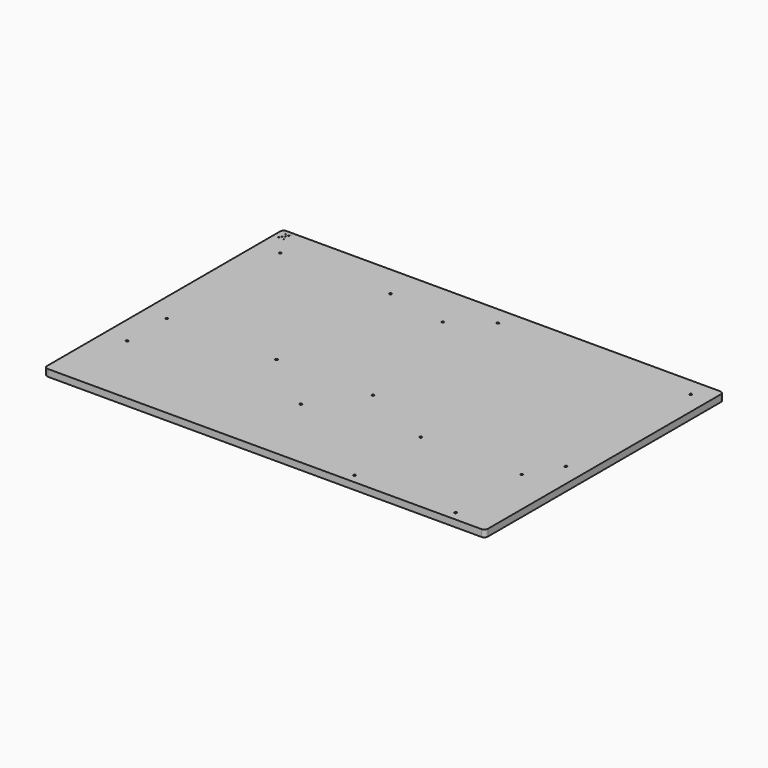
from build123d import *

# Parameters (mm, degrees)
F0_W         = 609.6
F0_H         = 412.75
F1_DEPTH     = 9.525
F2_R         = 1.5875
F3_DEPTH     = 25.4
F5_D         = 3.175
F7_D         = 3.175
F8_R         = 5.08
F9_TEXT_SIZE = 17.3569139507
F10_DEPTH    = 0.254


# Not quite as in the source:
# - Text() gives the source's letters only with a copy of the font that has no kerning and outlines rounded to 1/6400 em; it was checked with that copy


with BuildPart() as f1:
    # F0 (on Top) → F1 (new body)
    with BuildSketch(Plane.XY):
        with Locations((3.2237693667, 74.4166416769)):
            Rectangle(F0_W, F0_H)
    extrude(amount=F1_DEPTH)

    # F2 (on face) → F3 (cut)
    with BuildSketch(Plane.XY.offset(9.525)):
        with Locations((-269.8262306333, 236.3416416769)):
            Circle(F2_R)
        with Locations((-269.8262306333, 40.2536416769)):
            Circle(F2_R)
        with Locations((-270.5882306333, -27.2341583231)):
            Circle(F2_R)
        with Locations((-117.4262306333, 236.3416416769)):
            Circle(F2_R)
        with Locations((-117.4262306333, 39.4916416769)):
            Circle(F2_R)
        with Locations((-31.7012306333, -25.7101583231)):
            Circle(F2_R)
        with Locations((-32.0822306333, 220.1872416769)):
            Circle(F2_R)
    extrude(amount=-F3_DEPTH, mode=Mode.SUBTRACT)

    # F5 (through all)
    with Locations(Plane.XY.offset(9.525)):
        with Locations((117.5237693667, -4.9583583231), (257.2237693667, -4.9583583231), (257.2237693667, -119.2583583231), (117.5237693667, -119.2583583231)):
            Hole(F5_D / 2)

    # F7 (through all)
    with Locations(Plane.XY.offset(9.525)):
        with Locations((15.9237693667, 255.3916416769), (282.6237693667, 255.3916416769), (282.6237693667, 39.4916416769), (15.9237693667, 39.4916416769)):
            Hole(F7_D / 2)

    # F8
    f8_edges = [f1.edges().sort_by_distance(p)[0] for p in [
        (-301.576231, -131.958358, 4.7625),
        (-301.576231, 280.791642, 4.7625),
        (308.023769, 280.791642, 4.7625),
        (308.023769, -131.958358, 4.7625),
    ]]
    fillet(f8_edges, radius=F8_R)

    # F9 (on face) → F10 (join)
    with BuildSketch(Plane.XY.offset(9.525)):
        with Locations((-295.6899702549, 263.8282775879)):
            Text('X', F9_TEXT_SIZE, font='Open Sans', text_align=(TextAlign.LEFT, TextAlign.BOTTOM))
    extrude(amount=F10_DEPTH)


solid = f1.part
